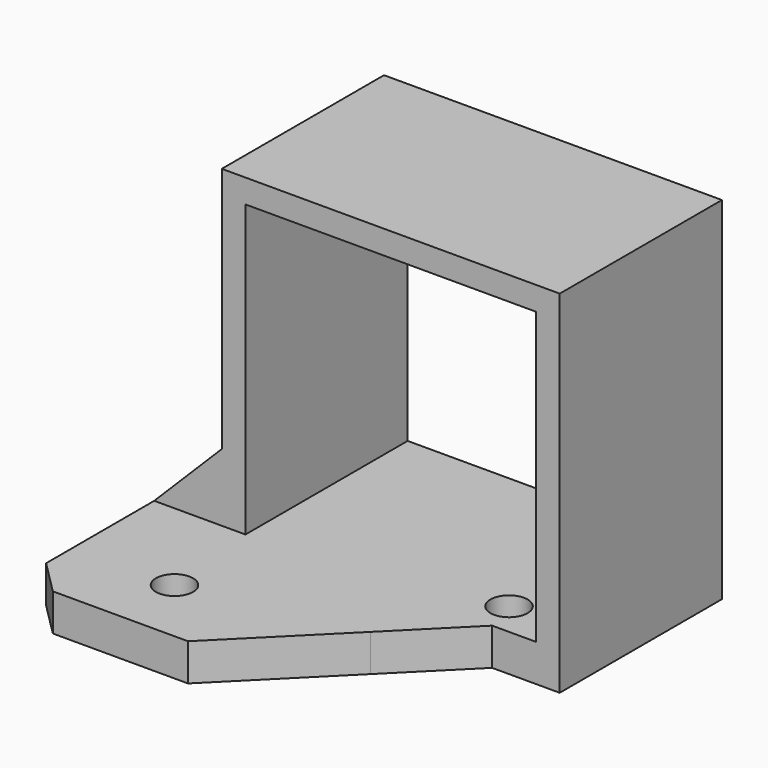
from build123d import *

# Parameters (mm, degrees)
F0_W          = 50
F0_H          = 52
F2_DEPTH      = 30
F1_W          = 43
F1_H          = 43
F3_DEPTH      = 30
F5_W          = 40
F5_H          = 30
F6_DEPTH      = 5.5
F4_W          = 10
F4_H          = 5.5
F7_DEPTH      = 20
F8_R          = 1.5
F9_DEPTH      = 25
F10_R         = 2.75
F11_DEPTH     = 3
F12_T1_DEPTH  = 5.5
F12_T6_DEPTH  = 5.5
F12_T11_DEPTH = 5
F12_T17_DEPTH = 31.2168298797
F12_T22_DEPTH = 30.7168298797
F13_SIZE      = 14.99999
F14_SIZE      = 5
F15_SIZE      = 5


# Not quite as in the source:
# - a fillet or chamfer that OpenCascade refuses, or shapes differently, is made with other operations: its cross-section is extruded or revolved along the edge and cut away or added
# - a fillet or chamfer is up to 0.001 mm smaller than in the source, because OpenCascade refuses the exact size


with BuildPart() as f2:
    # F0 (on Front) → F2 (new body)
    with BuildSketch(Plane.XZ):
        with Locations((0, -1)):
            Rectangle(F0_W, F0_H)
    extrude(amount=F2_DEPTH)

    # F1 (on face) → F3 (cut)
    with BuildSketch(Plane.XZ):
        Rectangle(F1_W, F1_H)
    extrude(amount=F3_DEPTH, mode=Mode.SUBTRACT)

    # F5 (on face) → F6 (join)
    with BuildSketch(Plane.XY.offset(-21.5)):
        with Locations((-15, -40)):
            Rectangle(F5_W, F5_H)
    extrude(amount=-F6_DEPTH)

    # F4 (on face) → F7 (join)
    with BuildSketch(Plane.XZ.offset(30)):
        with Locations((-20, -24.25)):
            Rectangle(F4_W, F4_H)
    extrude(amount=F7_DEPTH)

    # F8 (on face) → F9 (cut)
    with BuildSketch(Plane.XY.offset(-21.5)):
        with Locations((-20, -45)):
            Circle(F8_R)
        with Locations((13.5, -25)):
            Circle(F8_R)
    extrude(amount=-F9_DEPTH, mode=Mode.SUBTRACT)

    # F10 (on face) → F11 (cut)
    with BuildSketch(Plane.XY.offset(-21.5)):
        with Locations((-20, -45)):
            Circle(F10_R)
        with Locations((13.5, -25)):
            Circle(F10_R)
    extrude(amount=-F11_DEPTH, mode=Mode.SUBTRACT)

    # F12: chamfer of 10 on 3 edges, made by hand

    # F12_s2 → F12_t1 (join)
    with BuildSketch(Plane.XY.offset(-27)):
        Polygon((15, -30), (5, -40), (5, -30), align=None)
    extrude(amount=F12_T1_DEPTH)


with BuildPart() as f12_tool4:
    # F12_s5 → F12_t6 (new body)
    with BuildSketch(Plane.XY.offset(-27)):
        Polygon((-25, -15), (-35, -25), (-25, -25), align=None)
    extrude(amount=F12_T6_DEPTH)

    split(bisect_by=Plane.YZ.offset(-35), keep=Keep.TOP)


with BuildPart() as f2_1:
    add(f2.part)

    # F12_t3: union F12_tool4
    add(f12_tool4.part)


with BuildPart() as f12_tool9:
    # F12_s10 → F12_t11 (new body)
    with BuildSketch(Plane.XZ.offset(25)):
        Polygon((-25, -11.5), (-35, -21.5), (-25, -21.5), align=None)
    extrude(amount=F12_T11_DEPTH)

    split(bisect_by=Plane.YZ.offset(-35), keep=Keep.TOP)


with BuildPart() as f2_2:
    add(f2_1.part)

    # F12_t8: union F12_tool9
    add(f12_tool9.part)


with BuildPart() as f12_tool15:
    # F12_s16 → F12_t17 (new body)
    with BuildSketch(Plane.XY.offset(-27)):
        Polygon((-25, -15), (-35, -25), (-25, -25), align=None)
    extrude(amount=F12_T17_DEPTH)

    split(bisect_by=Plane.XY.offset(-21.5), keep=Keep.TOP)

    split(bisect_by=Plane.YZ.offset(-35), keep=Keep.TOP)


with BuildPart() as f12_tool20:
    # F12_s21 → F12_t22 (new body)
    with BuildSketch(Plane.XZ.offset(-0.7168298797)):
        Polygon((-25, -11.5), (-35, -21.5), (-25, -21.5), align=None)
    extrude(amount=F12_T22_DEPTH)

    split(bisect_by=Plane.XZ, keep=Keep.TOP)

    split(bisect_by=Plane.XZ.offset(25), keep=Keep.BOTTOM)

    split(bisect_by=Plane.YZ.offset(-35), keep=Keep.TOP)


with BuildPart() as f12_tool15_1:
    add(f12_tool15.part)

    # F12_t26: intersect F12_tool20
    add(f12_tool20.part, mode=Mode.INTERSECT)


with BuildPart() as f2_3:
    add(f2_2.part)

    # F12_t13: union F12_tool15
    add(f12_tool15_1.part)

    # F13 (size 15 in the source; OpenCascade refuses exactly that, so slightly less here)
    f13_edges = [f2_3.edges().sort_by_distance(p)[0] for p in [
        (5, -55, -24.25),
    ]]
    chamfer(f13_edges, length=F13_SIZE)

    # F14
    f14_edges = [f2_3.edges().sort_by_distance(p)[0] for p in [
        (-35, -55, -24.25),
    ]]
    chamfer(f14_edges, length=F14_SIZE)

    # F15
    f15_edges = [f2_3.edges().sort_by_distance(p)[0] for p in [
        (-35, -25, -24.25),
    ]]
    chamfer(f15_edges, length=F15_SIZE)


solid = f2_3.part
